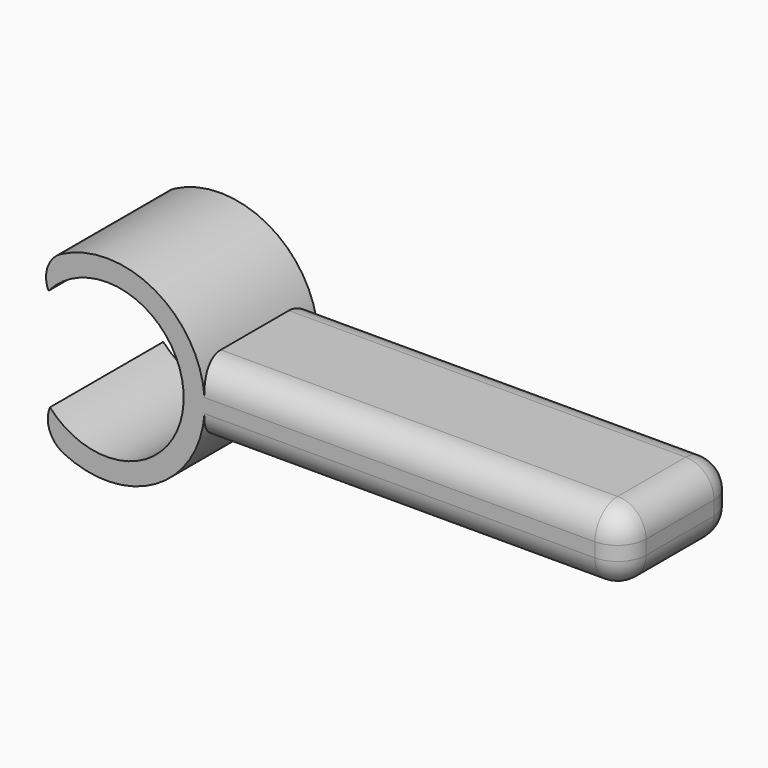
from build123d import *

# Parameters (mm, degrees)
F1_DEPTH    = 25.4
F2_F1_R     = 5.08
F2_F2_R     = 5.08
F2_F3_R     = 5.08
F2_F4_R     = 5.08
F5_T1_DEPTH = 57.4399599705
F5_T3_DEPTH = 60.5847169717


# Not quite as in the source:
# - a fillet or chamfer that OpenCascade refuses, or shapes differently, is made with other operations: its cross-section is extruded or revolved along the edge and cut away or added
# - a feature of the source that left no trace in its solid (it failed there, or was rolled back) is left out


with BuildPart() as f1:
    # F0 (on Front) → F1 (new body)
    with BuildSketch(Plane.XZ):
        with BuildLine():
            ThreePointArc((19.913375901, 8.2747844221), (44.1487619553, -0.5270852778), (20.1739600729, -10.0158007924))
            Line((20.1739600729, -10.0158007924), (17.0700166839, -12.2068939621))
            ThreePointArc((17.0700166839, -12.2068939621), (33.3560783856, -18.0313258742), (46.7383854464, -7.0735126536))
            Line((46.7383854464, -7.0735126536), (46.7383854464, 5.6264873464))
            ThreePointArc((46.7383854464, 5.6264873464), (33.4251988827, 16.5721987148), (17.1621920022, 10.8656988202))
            Line((17.1621920022, 10.8656988202), (19.913375901, 8.2747844221))
        make_face()
        with BuildLine():
            Line((46.7383854464, 5.6264873464), (46.7383854464, -7.0735126536))
            ThreePointArc((46.7383854464, -7.0735126536), (47.9263685939, -0.7235126536), (46.7383854464, 5.6264873464))
        make_face()
        with BuildLine():
            ThreePointArc((46.7383854464, 5.6264873464), (47.9263685939, -0.7235126536), (46.7383854464, -7.0735126536))
            Line((46.7383854464, -7.0735126536), (122.9383854464, -7.0735126536))
            Line((122.9383854464, -7.0735126536), (122.9383854464, 5.6264873464))
            Line((122.9383854464, 5.6264873464), (46.7383854464, 5.6264873464))
        make_face()
    extrude(amount=F1_DEPTH)

    # F2: fillet of radius 5.08 on 4 edges, made by hand

    # F2_f1
    f2_f1_edges = [f1.edges().sort_by_distance(p)[0] for p in [
        (122.9383854464, -12.7, -7.0735126536),
    ]]
    fillet(f2_f1_edges, radius=F2_F1_R)

    # F2_f2
    f2_f2_edges = [f1.edges().sort_by_distance(p)[0] for p in [
        (122.9383854464, -12.7, 5.6264873464),
    ]]
    fillet(f2_f2_edges, radius=F2_F2_R)

    # F2_f3
    f2_f3_edges = [f1.edges().sort_by_distance(p)[0] for p in [
        (122.9383854464, 0, -0.7235126536),
    ]]
    fillet(f2_f3_edges, radius=F2_F3_R)

    # F2_f4
    f2_f4_edges = [f1.edges().sort_by_distance(p)[0] for p in [
        (122.9383854464, -25.4, -0.7235126536),
    ]]
    fillet(f2_f4_edges, radius=F2_F4_R)

    # F5: fillet of radius 5.08 on 2 edges, made by hand

    # F5_s2 → F5_t1 (cut)
    with BuildSketch(Plane.XZ.offset(-16.0199799852)):
        with BuildLine():
            ThreePointArc((19.913375901, 8.2747844221), (19.7615867452, 12.0028035456), (22.1975397768, 14.8289846016))
            ThreePointArc((22.1975397768, 14.8289846016), (19.4976030488, 13.0789063368), (17.1621920022, 10.8656988202))
            Line((17.1621920022, 10.8656988202), (19.913375901, 8.2747844221))
        make_face()
    extrude(amount=F5_T1_DEPTH, mode=Mode.SUBTRACT)

    # F5_s4 → F5_t3 (cut)
    with BuildSketch(Plane.XZ.offset(-17.5923584858)):
        with BuildLine():
            ThreePointArc((22.6439130786, -16.5022695354), (20.1284364115, -13.7466310122), (20.1739600729, -10.0158007924))
            Line((20.1739600729, -10.0158007924), (17.0700166839, -12.2068939621))
            ThreePointArc((17.0700166839, -12.2068939621), (19.6396592089, -14.6365685699), (22.6439130786, -16.5022695354))
        make_face()
    extrude(amount=F5_T3_DEPTH, mode=Mode.SUBTRACT)


solid = f1.part
